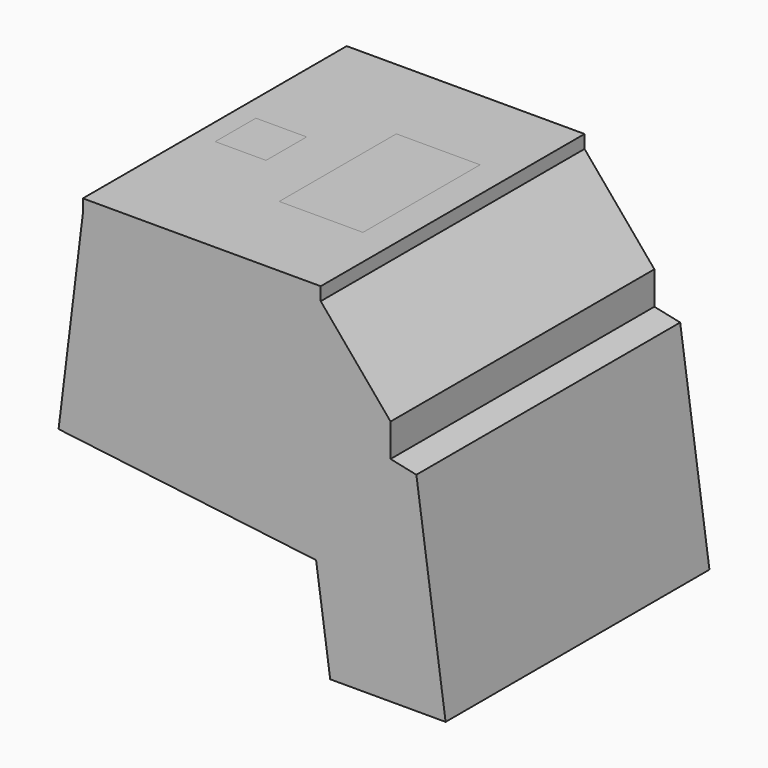
from build123d import *

# Parameters (mm, degrees)
F1_DEPTH       = 500
F2_W           = 160
F2_H           = 160
F3_DEPTH       = 40
F4_W           = 260
F4_H           = 450
F5_DEPTH       = 40
F6_T           = -3
F8_DEPTH       = 497
F8_DEPTH_BACK  = 497
F9_W           = 721.3165694991
F9_H           = 1000
F9_W_2         = 160
F9_H_2         = 160
F9_W_3         = 260
F9_H_3         = 450
F10_DEPTH      = 40
F12_DEPTH      = 497
F12_DEPTH_BACK = 497
F13_W          = 20
F13_H          = 100
F14_DEPTH      = 20
F16_DEPTH      = 497
F16_DEPTH_BACK = 497
F17_W          = 20
F17_H          = 100
F18_DEPTH      = 20
F21_DEPTH      = 500
F21_DEPTH_BACK = 500
F23_DEPTH      = 500
F23_DEPTH_BACK = 500
F25_DEPTH      = 500
F25_DEPTH_BACK = 500


# Not quite as in the source:
# - a feature names something its author has since deleted; it is built from what else it names


with BuildPart() as f1:
    # F0 (on Front) → F1 (new body, symmetric)
    with BuildSketch(Plane.XZ):
        Polygon((207.2595909262, -195.8861873539), (250, -500), (600, -500), (511.3165694991, 131.0153962632), (433.0647614404, 147.6483315286), (433.0647614404, 247.6483315286), (221.3165694991, 500), (-500, 500), (-573.6707365417, -100), align=None)
    extrude(amount=F1_DEPTH, both=True)

    # F2 (on face) → F3 (join)
    with BuildSketch(Plane.XY.offset(500)):
        with Locations((-360, 0)):
            Rectangle(F2_W, F2_H)
    extrude(amount=F3_DEPTH)

    # F4 (on face) → F5 (join)
    with BuildSketch(Plane.XY.offset(500)):
        Rectangle(F4_W, F4_H)
    extrude(amount=F5_DEPTH)

    # F6
    f6_openings = [f1.faces().sort_by_distance(p)[0] for p in [
        (-360, 0, 540),
        (0, 0, 540),
        (425, 0, -500),
    ]]
    offset(amount=F6_T, openings=f6_openings, kind=Kind.INTERSECTION)

    # F7 (on Front) → F8 (join, two sides)
    with BuildSketch(Plane.XZ) as f8_sk:
        Polygon((-272.9249017454, 497), (-283, 497), (-303.5681516407, 329.485847655), (-412.7482283212, 342.8914754296), (-413.9669217553, 332.9660139132), (-294.8613835583, 318.3416927046), align=None)
        Polygon((-354.5284905895, 265.2173027142), (-523.2613363685, 285.9350910931), (-524.4800298025, 276.0096295767), (-365.6726455399, 256.5105346318), (-368.110032408, 236.659611599), (-358.1845708916, 235.440918165), align=None)
        Polygon((-201.4627454091, 34.8461290566), (-548.8538984836, 77.5003992484), (-550.0725919176, 67.574937732), (-212.6069003596, 26.1393609742), (-215.0442872277, 6.2884379414), (-205.1188257113, 5.0697445073), align=None)
        Polygon((488.6612553675, -227.4154376833), (478.3856614799, -226.1537533998), (516.8722415573, -500), (526.9705172824, -500), align=None)
    extrude(amount=-F8_DEPTH)
    extrude(f8_sk.sketch, amount=F8_DEPTH_BACK)

    # F9 (on face) → F10 (join, through all)
    with BuildSketch(Plane.XY.offset(500)):
        with Locations((-139.3417152504, 0)):
            Rectangle(F9_W, F9_H)
        with Locations((-360, 0)):
            Rectangle(F9_W_2, F9_H_2, mode=Mode.SUBTRACT)
        Rectangle(F9_W_3, F9_H_3, mode=Mode.SUBTRACT)
    extrude(amount=F10_DEPTH)


with BuildPart() as f12:
    # F11 (on Front) → F12 (new body, two sides)
    with BuildSketch(Plane.XZ) as f12_sk:
        Polygon((-385.0238507034, -69.764904294), (-382.5864638353, -49.9139812612), (399.8078768519, -145.9799268354), (476.9939304703, -216.2510727124), (478.38566148, -226.1537533998), (488.6612553675, -227.4154376833), (486.3943923443, -211.2858691632), (391.3943923443, -124.7966843253), (-400, -27.6256713603), (-404.8747737362, -67.3275174259), align=None)
    extrude(amount=F12_DEPTH)
    extrude(f12_sk.sketch, amount=-F12_DEPTH_BACK)

    # F13 (on face) → F14 (cut, through all)
    with BuildSketch(Plane(origin=(-9.2824821361, 0, -75.5997502283), x_dir=(0.9925461516, 0, -0.1218693434), z_dir=(0.1218693434, 0, 0.9925461516))):
        with Locations((370, 420)):
            Rectangle(F13_W, F13_H)
        with Locations((370, 280)):
            Rectangle(F13_W, F13_H)
        with Locations((370, 140)):
            Rectangle(F13_W, F13_H)
        with Locations((370, 0)):
            Rectangle(F13_W, F13_H)
        with Locations((370, -140)):
            Rectangle(F13_W, F13_H)
        with Locations((370, -280)):
            Rectangle(F13_W, F13_H)
        with Locations((370, -420)):
            Rectangle(F13_W, F13_H)
        with Locations((320, 420)):
            Rectangle(F13_W, F13_H)
        with Locations((320, 280)):
            Rectangle(F13_W, F13_H)
        with Locations((320, 140)):
            Rectangle(F13_W, F13_H)
        with Locations((320, 0)):
            Rectangle(F13_W, F13_H)
        with Locations((320, -140)):
            Rectangle(F13_W, F13_H)
        with Locations((320, -280)):
            Rectangle(F13_W, F13_H)
        with Locations((320, -420)):
            Rectangle(F13_W, F13_H)
        with Locations((270, 420)):
            Rectangle(F13_W, F13_H)
        with Locations((270, 280)):
            Rectangle(F13_W, F13_H)
        with Locations((270, 140)):
            Rectangle(F13_W, F13_H)
        with Locations((270, 0)):
            Rectangle(F13_W, F13_H)
        with Locations((270, -140)):
            Rectangle(F13_W, F13_H)
        with Locations((270, -280)):
            Rectangle(F13_W, F13_H)
        with Locations((270, -420)):
            Rectangle(F13_W, F13_H)
        with Locations((220, 420)):
            Rectangle(F13_W, F13_H)
        with Locations((220, 280)):
            Rectangle(F13_W, F13_H)
        with Locations((220, 140)):
            Rectangle(F13_W, F13_H)
        with Locations((220, 0)):
            Rectangle(F13_W, F13_H)
        with Locations((220, -140)):
            Rectangle(F13_W, F13_H)
        with Locations((220, -280)):
            Rectangle(F13_W, F13_H)
        with Locations((220, -420)):
            Rectangle(F13_W, F13_H)
        with Locations((170, 420)):
            Rectangle(F13_W, F13_H)
        with Locations((170, 280)):
            Rectangle(F13_W, F13_H)
        with Locations((170, 140)):
            Rectangle(F13_W, F13_H)
        with Locations((170, 0)):
            Rectangle(F13_W, F13_H)
        with Locations((170, -140)):
            Rectangle(F13_W, F13_H)
        with Locations((170, -280)):
            Rectangle(F13_W, F13_H)
        with Locations((170, -420)):
            Rectangle(F13_W, F13_H)
        with Locations((120, 420)):
            Rectangle(F13_W, F13_H)
        with Locations((120, 280)):
            Rectangle(F13_W, F13_H)
        with Locations((120, 140)):
            Rectangle(F13_W, F13_H)
        with Locations((120, 0)):
            Rectangle(F13_W, F13_H)
        with Locations((120, -140)):
            Rectangle(F13_W, F13_H)
        with Locations((120, -280)):
            Rectangle(F13_W, F13_H)
        with Locations((120, -420)):
            Rectangle(F13_W, F13_H)
        with Locations((70, 420)):
            Rectangle(F13_W, F13_H)
        with Locations((70, 280)):
            Rectangle(F13_W, F13_H)
        with Locations((70, 140)):
            Rectangle(F13_W, F13_H)
        with Locations((70, 0)):
            Rectangle(F13_W, F13_H)
        with Locations((70, -140)):
            Rectangle(F13_W, F13_H)
        with Locations((70, -280)):
            Rectangle(F13_W, F13_H)
        with Locations((70, -420)):
            Rectangle(F13_W, F13_H)
        with Locations((20, 420)):
            Rectangle(F13_W, F13_H)
        with Locations((20, 280)):
            Rectangle(F13_W, F13_H)
        with Locations((20, 140)):
            Rectangle(F13_W, F13_H)
        with Locations((20, 0)):
            Rectangle(F13_W, F13_H)
        with Locations((20, -140)):
            Rectangle(F13_W, F13_H)
        with Locations((20, -280)):
            Rectangle(F13_W, F13_H)
        with Locations((20, -420)):
            Rectangle(F13_W, F13_H)
        with Locations((-30, 420)):
            Rectangle(F13_W, F13_H)
        with Locations((-30, 280)):
            Rectangle(F13_W, F13_H)
        with Locations((-30, 140)):
            Rectangle(F13_W, F13_H)
        with Locations((-30, 0)):
            Rectangle(F13_W, F13_H)
        with Locations((-30, -140)):
            Rectangle(F13_W, F13_H)
        with Locations((-30, -280)):
            Rectangle(F13_W, F13_H)
        with Locations((-30, -420)):
            Rectangle(F13_W, F13_H)
        with Locations((-80, 420)):
            Rectangle(F13_W, F13_H)
        with Locations((-80, 280)):
            Rectangle(F13_W, F13_H)
        with Locations((-80, 140)):
            Rectangle(F13_W, F13_H)
        with Locations((-80, 0)):
            Rectangle(F13_W, F13_H)
        with Locations((-80, -140)):
            Rectangle(F13_W, F13_H)
        with Locations((-80, -280)):
            Rectangle(F13_W, F13_H)
        with Locations((-80, -420)):
            Rectangle(F13_W, F13_H)
        with Locations((-130, 420)):
            Rectangle(F13_W, F13_H)
        with Locations((-130, 280)):
            Rectangle(F13_W, F13_H)
        with Locations((-130, 140)):
            Rectangle(F13_W, F13_H)
        with Locations((-130, 0)):
            Rectangle(F13_W, F13_H)
        with Locations((-130, -140)):
            Rectangle(F13_W, F13_H)
        with Locations((-130, -280)):
            Rectangle(F13_W, F13_H)
        with Locations((-130, -420)):
            Rectangle(F13_W, F13_H)
        with Locations((-180, 420)):
            Rectangle(F13_W, F13_H)
        with Locations((-180, 280)):
            Rectangle(F13_W, F13_H)
        with Locations((-180, 140)):
            Rectangle(F13_W, F13_H)
        with Locations((-180, 0)):
            Rectangle(F13_W, F13_H)
        with Locations((-180, -140)):
            Rectangle(F13_W, F13_H)
        with Locations((-180, -280)):
            Rectangle(F13_W, F13_H)
        with Locations((-180, -420)):
            Rectangle(F13_W, F13_H)
        with Locations((-230, 420)):
            Rectangle(F13_W, F13_H)
        with Locations((-230, 280)):
            Rectangle(F13_W, F13_H)
        with Locations((-230, 140)):
            Rectangle(F13_W, F13_H)
        with Locations((-230, 0)):
            Rectangle(F13_W, F13_H)
        with Locations((-230, -140)):
            Rectangle(F13_W, F13_H)
        with Locations((-230, -280)):
            Rectangle(F13_W, F13_H)
        with Locations((-230, -420)):
            Rectangle(F13_W, F13_H)
        with Locations((-280, 420)):
            Rectangle(F13_W, F13_H)
        with Locations((-280, 280)):
            Rectangle(F13_W, F13_H)
        with Locations((-280, 140)):
            Rectangle(F13_W, F13_H)
        with Locations((-280, 0)):
            Rectangle(F13_W, F13_H)
        with Locations((-280, -140)):
            Rectangle(F13_W, F13_H)
        with Locations((-280, -280)):
            Rectangle(F13_W, F13_H)
        with Locations((-280, -420)):
            Rectangle(F13_W, F13_H)
        with Locations((-330, 420)):
            Rectangle(F13_W, F13_H)
        with Locations((-330, 280)):
            Rectangle(F13_W, F13_H)
        with Locations((-330, 140)):
            Rectangle(F13_W, F13_H)
        with Locations((-330, 0)):
            Rectangle(F13_W, F13_H)
        with Locations((-330, -140)):
            Rectangle(F13_W, F13_H)
        with Locations((-330, -280)):
            Rectangle(F13_W, F13_H)
        with Locations((-330, -420)):
            Rectangle(F13_W, F13_H)
    extrude(amount=-F14_DEPTH, mode=Mode.SUBTRACT)


with BuildPart() as f16:
    # F15 (on Front) → F16 (new body, two sides)
    with BuildSketch(Plane.XZ) as f16_sk:
        Polygon((-481.4627454091, 149.8265921461), (-483.9001322772, 129.9756691133), (376.482267621, 24.3339939332), (454.9584935667, -40.7147154111), (461.3401583867, -33.015731444), (366.3401583867, 45.7294848713), align=None)
    extrude(amount=F16_DEPTH)
    extrude(f16_sk.sketch, amount=-F16_DEPTH_BACK)

    # F17 (on face) → F18 (cut, through all)
    with BuildSketch(Plane(origin=(10.9724160028, 0, 89.363157079), x_dir=(0.9925461516, 0, -0.1218693434), z_dir=(0.1218693434, 0, 0.9925461516))):
        with Locations((305.9516142895, 420)):
            Rectangle(F17_W, F17_H)
        with Locations((305.9516142895, 280)):
            Rectangle(F17_W, F17_H)
        with Locations((305.9516142895, 140)):
            Rectangle(F17_W, F17_H)
        with Locations((305.9516142895, 0)):
            Rectangle(F17_W, F17_H)
        with Locations((305.9516142895, -140)):
            Rectangle(F17_W, F17_H)
        with Locations((305.9516142895, -280)):
            Rectangle(F17_W, F17_H)
        with Locations((305.9516142895, -420)):
            Rectangle(F17_W, F17_H)
        with Locations((255.9516142895, 420)):
            Rectangle(F17_W, F17_H)
        with Locations((255.9516142895, 280)):
            Rectangle(F17_W, F17_H)
        with Locations((255.9516142895, 140)):
            Rectangle(F17_W, F17_H)
        with Locations((255.9516142895, 0)):
            Rectangle(F17_W, F17_H)
        with Locations((255.9516142895, -140)):
            Rectangle(F17_W, F17_H)
        with Locations((255.9516142895, -280)):
            Rectangle(F17_W, F17_H)
        with Locations((255.9516142895, -420)):
            Rectangle(F17_W, F17_H)
        with Locations((205.9516142895, 420)):
            Rectangle(F17_W, F17_H)
        with Locations((205.9516142895, 280)):
            Rectangle(F17_W, F17_H)
        with Locations((205.9516142895, 140)):
            Rectangle(F17_W, F17_H)
        with Locations((205.9516142895, 0)):
            Rectangle(F17_W, F17_H)
        with Locations((205.9516142895, -140)):
            Rectangle(F17_W, F17_H)
        with Locations((205.9516142895, -280)):
            Rectangle(F17_W, F17_H)
        with Locations((205.9516142895, -420)):
            Rectangle(F17_W, F17_H)
        with Locations((155.9516142895, 420)):
            Rectangle(F17_W, F17_H)
        with Locations((155.9516142895, 280)):
            Rectangle(F17_W, F17_H)
        with Locations((155.9516142895, 140)):
            Rectangle(F17_W, F17_H)
        with Locations((155.9516142895, 0)):
            Rectangle(F17_W, F17_H)
        with Locations((155.9516142895, -140)):
            Rectangle(F17_W, F17_H)
        with Locations((155.9516142895, -280)):
            Rectangle(F17_W, F17_H)
        with Locations((155.9516142895, -420)):
            Rectangle(F17_W, F17_H)
        with Locations((105.9516142895, 420)):
            Rectangle(F17_W, F17_H)
        with Locations((105.9516142895, 280)):
            Rectangle(F17_W, F17_H)
        with Locations((105.9516142895, 140)):
            Rectangle(F17_W, F17_H)
        with Locations((105.9516142895, 0)):
            Rectangle(F17_W, F17_H)
        with Locations((105.9516142895, -140)):
            Rectangle(F17_W, F17_H)
        with Locations((105.9516142895, -280)):
            Rectangle(F17_W, F17_H)
        with Locations((105.9516142895, -420)):
            Rectangle(F17_W, F17_H)
        with Locations((55.9516142895, 420)):
            Rectangle(F17_W, F17_H)
        with Locations((55.9516142895, 280)):
            Rectangle(F17_W, F17_H)
        with Locations((55.9516142895, 140)):
            Rectangle(F17_W, F17_H)
        with Locations((55.9516142895, 0)):
            Rectangle(F17_W, F17_H)
        with Locations((55.9516142895, -140)):
            Rectangle(F17_W, F17_H)
        with Locations((55.9516142895, -280)):
            Rectangle(F17_W, F17_H)
        with Locations((55.9516142895, -420)):
            Rectangle(F17_W, F17_H)
        with Locations((5.9516142895, 420)):
            Rectangle(F17_W, F17_H)
        with Locations((5.9516142895, 280)):
            Rectangle(F17_W, F17_H)
        with Locations((5.9516142895, 140)):
            Rectangle(F17_W, F17_H)
        with Locations((5.9516142895, 0)):
            Rectangle(F17_W, F17_H)
        with Locations((5.9516142895, -140)):
            Rectangle(F17_W, F17_H)
        with Locations((5.9516142895, -280)):
            Rectangle(F17_W, F17_H)
        with Locations((5.9516142895, -420)):
            Rectangle(F17_W, F17_H)
        with Locations((-44.0483857105, 420)):
            Rectangle(F17_W, F17_H)
        with Locations((-44.0483857105, 280)):
            Rectangle(F17_W, F17_H)
        with Locations((-44.0483857105, 140)):
            Rectangle(F17_W, F17_H)
        with Locations((-44.0483857105, 0)):
            Rectangle(F17_W, F17_H)
        with Locations((-44.0483857105, -140)):
            Rectangle(F17_W, F17_H)
        with Locations((-44.0483857105, -280)):
            Rectangle(F17_W, F17_H)
        with Locations((-44.0483857105, -420)):
            Rectangle(F17_W, F17_H)
        with Locations((-94.0483857105, 420)):
            Rectangle(F17_W, F17_H)
        with Locations((-94.0483857105, 280)):
            Rectangle(F17_W, F17_H)
        with Locations((-94.0483857105, 140)):
            Rectangle(F17_W, F17_H)
        with Locations((-94.0483857105, 0)):
            Rectangle(F17_W, F17_H)
        with Locations((-94.0483857105, -140)):
            Rectangle(F17_W, F17_H)
        with Locations((-94.0483857105, -280)):
            Rectangle(F17_W, F17_H)
        with Locations((-94.0483857105, -420)):
            Rectangle(F17_W, F17_H)
        with Locations((-144.0483857105, 420)):
            Rectangle(F17_W, F17_H)
        with Locations((-144.0483857105, 280)):
            Rectangle(F17_W, F17_H)
        with Locations((-144.0483857105, 140)):
            Rectangle(F17_W, F17_H)
        with Locations((-144.0483857105, 0)):
            Rectangle(F17_W, F17_H)
        with Locations((-144.0483857105, -140)):
            Rectangle(F17_W, F17_H)
        with Locations((-144.0483857105, -280)):
            Rectangle(F17_W, F17_H)
        with Locations((-144.0483857105, -420)):
            Rectangle(F17_W, F17_H)
        with Locations((-194.0483857105, 420)):
            Rectangle(F17_W, F17_H)
        with Locations((-194.0483857105, 280)):
            Rectangle(F17_W, F17_H)
        with Locations((-194.0483857105, 140)):
            Rectangle(F17_W, F17_H)
        with Locations((-194.0483857105, 0)):
            Rectangle(F17_W, F17_H)
        with Locations((-194.0483857105, -140)):
            Rectangle(F17_W, F17_H)
        with Locations((-194.0483857105, -280)):
            Rectangle(F17_W, F17_H)
        with Locations((-194.0483857105, -420)):
            Rectangle(F17_W, F17_H)
        with Locations((-244.0483857105, 420)):
            Rectangle(F17_W, F17_H)
        with Locations((-244.0483857105, 280)):
            Rectangle(F17_W, F17_H)
        with Locations((-244.0483857105, 140)):
            Rectangle(F17_W, F17_H)
        with Locations((-244.0483857105, 0)):
            Rectangle(F17_W, F17_H)
        with Locations((-244.0483857105, -140)):
            Rectangle(F17_W, F17_H)
        with Locations((-244.0483857105, -280)):
            Rectangle(F17_W, F17_H)
        with Locations((-244.0483857105, -420)):
            Rectangle(F17_W, F17_H)
        with Locations((-294.0483857105, 420)):
            Rectangle(F17_W, F17_H)
        with Locations((-294.0483857105, 280)):
            Rectangle(F17_W, F17_H)
        with Locations((-294.0483857105, 140)):
            Rectangle(F17_W, F17_H)
        with Locations((-294.0483857105, 0)):
            Rectangle(F17_W, F17_H)
        with Locations((-294.0483857105, -140)):
            Rectangle(F17_W, F17_H)
        with Locations((-294.0483857105, -280)):
            Rectangle(F17_W, F17_H)
        with Locations((-294.0483857105, -420)):
            Rectangle(F17_W, F17_H)
        with Locations((-344.0483857105, 420)):
            Rectangle(F17_W, F17_H)
        with Locations((-344.0483857105, 280)):
            Rectangle(F17_W, F17_H)
        with Locations((-344.0483857105, 140)):
            Rectangle(F17_W, F17_H)
        with Locations((-344.0483857105, 0)):
            Rectangle(F17_W, F17_H)
        with Locations((-344.0483857105, -140)):
            Rectangle(F17_W, F17_H)
        with Locations((-344.0483857105, -280)):
            Rectangle(F17_W, F17_H)
        with Locations((-344.0483857105, -420)):
            Rectangle(F17_W, F17_H)
        with Locations((-394.0483857105, 420)):
            Rectangle(F17_W, F17_H)
        with Locations((-394.0483857105, 280)):
            Rectangle(F17_W, F17_H)
        with Locations((-394.0483857105, 140)):
            Rectangle(F17_W, F17_H)
        with Locations((-394.0483857105, 0)):
            Rectangle(F17_W, F17_H)
        with Locations((-394.0483857105, -140)):
            Rectangle(F17_W, F17_H)
        with Locations((-394.0483857105, -280)):
            Rectangle(F17_W, F17_H)
        with Locations((-394.0483857105, -420)):
            Rectangle(F17_W, F17_H)
        with Locations((-444.0483857105, 420)):
            Rectangle(F17_W, F17_H)
        with Locations((-444.0483857105, 280)):
            Rectangle(F17_W, F17_H)
        with Locations((-444.0483857105, 140)):
            Rectangle(F17_W, F17_H)
        with Locations((-444.0483857105, 0)):
            Rectangle(F17_W, F17_H)
        with Locations((-444.0483857105, -140)):
            Rectangle(F17_W, F17_H)
        with Locations((-444.0483857105, -280)):
            Rectangle(F17_W, F17_H)
        with Locations((-444.0483857105, -420)):
            Rectangle(F17_W, F17_H)
    extrude(amount=-F18_DEPTH, mode=Mode.SUBTRACT)


with BuildPart() as f21:
    # F20 (on Front) → F21 (new body, two sides)
    with BuildSketch(Plane.XZ) as f21_sk:
        Polygon((-573.6707365417, -100), (207.2595909262, -195.8861873539), (250, -500), (600, -500), (533.1830695603, -24.5728362066), (496.5417803544, -29.7224335762), (458.2517914345, -75.9163373788), (366.1665289132, 0.4128617443), (-547.5661099193, 112.6051225861), align=None)
    extrude(amount=F21_DEPTH)
    extrude(f21_sk.sketch, amount=-F21_DEPTH_BACK)

    # F26: cut F1, F12
    add(f1.part, mode=Mode.SUBTRACT)
    add(f12.part, mode=Mode.SUBTRACT)


with BuildPart() as f23:
    # F22 (on Front) → F23 (new body, two sides)
    with BuildSketch(Plane.XZ) as f23_sk:
        Polygon((-503.229665615, 177.6869795223), (376.6558970945, 69.6506170602), (496.5417803544, -29.7224335762), (533.1830695603, -24.5728362066), (511.3165694991, 131.0153962632), (433.0647614404, 147.6483315286), (433.0647614404, 247.6483315286), (221.3165694991, 500), (221.3165694991, 540), (-500, 540), (-500, 500), (-547.5661099193, 112.6051225861), (-511.7605196534, 108.2087489074), align=None)
    extrude(amount=F23_DEPTH)
    extrude(f23_sk.sketch, amount=-F23_DEPTH_BACK)

    # F27: cut F1
    add(f1.part, mode=Mode.SUBTRACT)


with BuildPart() as f25:
    # F24 (on Front) → F25 (new body, two sides)
    with BuildSketch(Plane.XZ) as f25_sk:
        Polygon((458.2517914345, -75.9163373788), (496.5417803544, -29.7224335762), (376.6558970945, 69.6506170602), (-503.229665615, 177.6869795223), (-511.7605196534, 108.2087489074), (366.1665289132, 0.4128617443), align=None)
    extrude(amount=F25_DEPTH)
    extrude(f25_sk.sketch, amount=-F25_DEPTH_BACK)

    # F28: cut F16, F1
    add(f16.part, mode=Mode.SUBTRACT)
    add(f1.part, mode=Mode.SUBTRACT)


solid = Compound([f1.part, f12.part, f16.part, f21.part, f23.part, f25.part])
